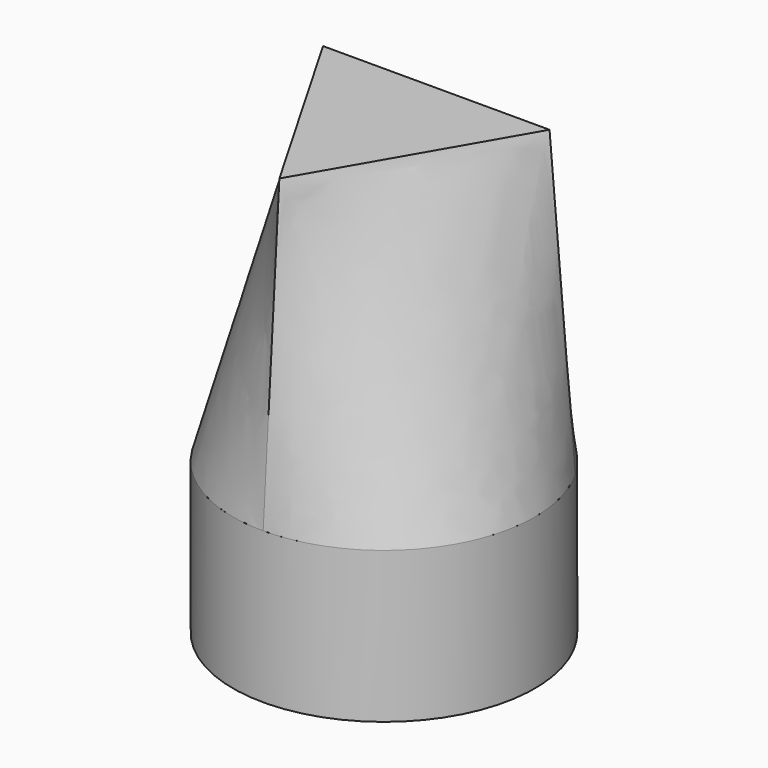
from build123d import *

# Parameters (mm, degrees)
F0_W = 50.8
F0_H = 50.8


# Not quite as in the source:
# - the arcs of a loft's sections are written as splines that run evenly, so that the points pair up as in the source's solid


with BuildPart() as f1:
    # F0 (on Front) → F1 (revolve)
    with BuildSketch(Plane.XZ):
        Rectangle(F0_W, F0_H)
    revolve(axis=Axis((25.4, 0, 0), (0, 0, -1)))

    # F3 (on offset) → F5 section 0
    with BuildSketch(Plane.XY.offset(127)):
        Polygon((63.5, 21.9970452561), (-12.7, 21.9970452561), (25.4, -43.9940905122), align=None)
    # F4 (on face) → F5 section 1
    with BuildSketch(Plane.XY.offset(25.4)):
        with BuildLine():
            add(Edge.make_bspline(
                [(69.3940905122, 25.4), (67.9163784122, 27.9594724362), (66.2147677676, 30.3896242866), (62.4153476533, 34.9175968576), (60.3175968576, 37.0153476533), (55.7896242866, 40.8147677676), (53.3594724362, 42.5163784122), (48.2405275638, 45.4718026123), (45.551813593, 46.7255705274), (39.9974329689, 48.7471997444), (37.1318520911, 49.5150298264), (31.3108027598, 50.5414378796), (28.3554242, 50.8), (22.4445758, 50.8), (19.4891972402, 50.5414378796), (13.6681479089, 49.5150298264), (10.8025670311, 48.7471997444), (5.248186407, 46.7255705274), (2.5594724362, 45.4718026123), (-2.5594724362, 42.5163784122), (-4.9896242866, 40.8147677676), (-9.5175968576, 37.0153476533), (-11.6153476533, 34.9175968576), (-15.4147677676, 30.3896242866), (-17.1163784122, 27.9594724362), (-18.5940905122, 25.4)],
                knots=[0, 0, 0, 0, 0.0833333333, 0.0833333333, 0.1666666667, 0.1666666667, 0.25, 0.25, 0.3333333333, 0.3333333333, 0.4166666667, 0.4166666667, 0.5, 0.5, 0.5833333333, 0.5833333333, 0.6666666667, 0.6666666667, 0.75, 0.75, 0.8333333333, 0.8333333333, 0.9166666667, 0.9166666667, 1, 1, 1, 1], degree=3))
            add(Edge.make_bspline(
                [(-18.5940905122, 25.4), (-20.0718026123, 22.8405275638), (-21.3255705274, 20.151813593), (-23.3471997444, 14.5974329689), (-24.1150298264, 11.7318520911), (-25.1414378796, 5.9108027598), (-25.4, 2.9554242), (-25.4, -2.9554242), (-25.1414378796, -5.9108027598), (-24.1150298264, -11.7318520911), (-23.3471997444, -14.5974329689), (-21.3255705274, -20.151813593), (-20.0718026123, -22.8405275638), (-17.1163784122, -27.9594724362), (-15.4147677676, -30.3896242866), (-11.6153476533, -34.9175968576), (-9.5175968576, -37.0153476533), (-4.9896242866, -40.8147677676), (-2.5594724362, -42.5163784122), (2.5594724362, -45.4718026123), (5.248186407, -46.7255705274), (10.8025670311, -48.7471997444), (13.6681479089, -49.5150298264), (19.4891972402, -50.5414378796), (22.4445758, -50.8), (25.4, -50.8)],
                knots=[0, 0, 0, 0, 0.0833333333, 0.0833333333, 0.1666666667, 0.1666666667, 0.25, 0.25, 0.3333333333, 0.3333333333, 0.4166666667, 0.4166666667, 0.5, 0.5, 0.5833333333, 0.5833333333, 0.6666666667, 0.6666666667, 0.75, 0.75, 0.8333333333, 0.8333333333, 0.9166666667, 0.9166666667, 1, 1, 1, 1], degree=3))
            add(Edge.make_bspline(
                [(25.4, -50.8), (28.3554242, -50.8), (31.3108027598, -50.5414378796), (37.1318520911, -49.5150298264), (39.9974329689, -48.7471997444), (45.551813593, -46.7255705274), (48.2405275638, -45.4718026123), (53.3594724362, -42.5163784122), (55.7896242866, -40.8147677676), (60.3175968576, -37.0153476533), (62.4153476533, -34.9175968576), (66.2147677676, -30.3896242866), (67.9163784122, -27.9594724362), (70.8718026123, -22.8405275638), (72.1255705274, -20.151813593), (74.1471997444, -14.5974329689), (74.9150298264, -11.7318520911), (75.9414378796, -5.9108027598), (76.2, -2.9554242), (76.2, 2.9554242), (75.9414378796, 5.9108027598), (74.9150298264, 11.7318520911), (74.1471997444, 14.5974329689), (72.1255705274, 20.151813593), (70.8718026123, 22.8405275638), (69.3940905122, 25.4)],
                knots=[0, 0, 0, 0, 0.0833333333, 0.0833333333, 0.1666666667, 0.1666666667, 0.25, 0.25, 0.3333333333, 0.3333333333, 0.4166666667, 0.4166666667, 0.5, 0.5, 0.5833333333, 0.5833333333, 0.6666666667, 0.6666666667, 0.75, 0.75, 0.8333333333, 0.8333333333, 0.9166666667, 0.9166666667, 1, 1, 1, 1], degree=3))
        make_face()
    loft(ruled=True)


solid = f1.part
